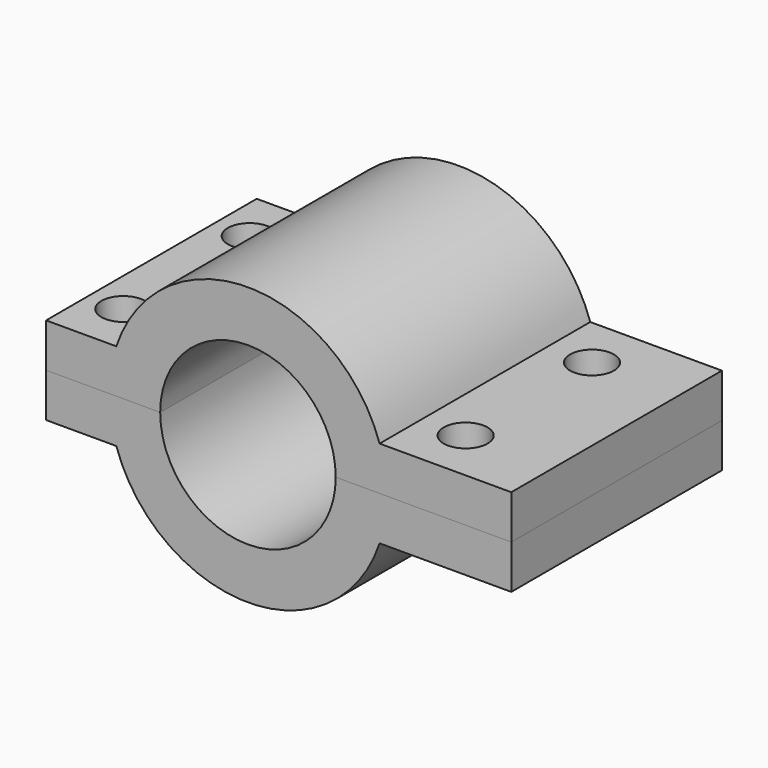
from build123d import *

# Parameters (mm, degrees)
F1_DEPTH = 38.1
F3_COUNT = 2
F4_R     = 3.175
F5_DEPTH = 25.4


with BuildPart() as f1:
    # F0 (on Front) → F1 (new body)
    with BuildSketch(Plane.XZ):
        with BuildLine():
            Line((-6.35, 0), (0, 0))
            Line((0, 0), (19.05, 0))
            Line((19.05, 0), (19.05, 6.35))
            Line((19.05, 6.35), (0, 6.35))
            ThreePointArc((0, 6.35), (-19.05, 20.0804631421), (-38.1, 6.35))
            Line((-38.1, 6.35), (-48.26, 6.35))
            Line((-48.26, 6.35), (-48.26, 0))
            Line((-48.26, 0), (-31.75, 0))
            ThreePointArc((-31.75, 0), (-19.05, 12.7), (-6.35, 0))
        make_face()
    extrude(amount=F1_DEPTH)


with BuildPart() as f3_1:
    # F3: instance of F1
    add(f1.part.rotate(Axis((-9.9853500724, -19.05, 0), (1, 0, 0)), 1 * 360 / F3_COUNT))


with BuildPart() as f1_1:
    add(f1.part)

    # F4 (on face) → F5 (cut)
    with BuildSketch(Plane.XY.offset(6.35)):
        with Locations((6.35, -7.62)):
            Circle(F4_R)
        with Locations((6.35, -30.48)):
            Circle(F4_R)
        with Locations((-43.18, -30.48)):
            Circle(F4_R)
        with Locations((-43.18, -7.62)):
            Circle(F4_R)
    extrude(amount=-F5_DEPTH, mode=Mode.SUBTRACT)


solid = Compound([f3_1.part, f1_1.part])
